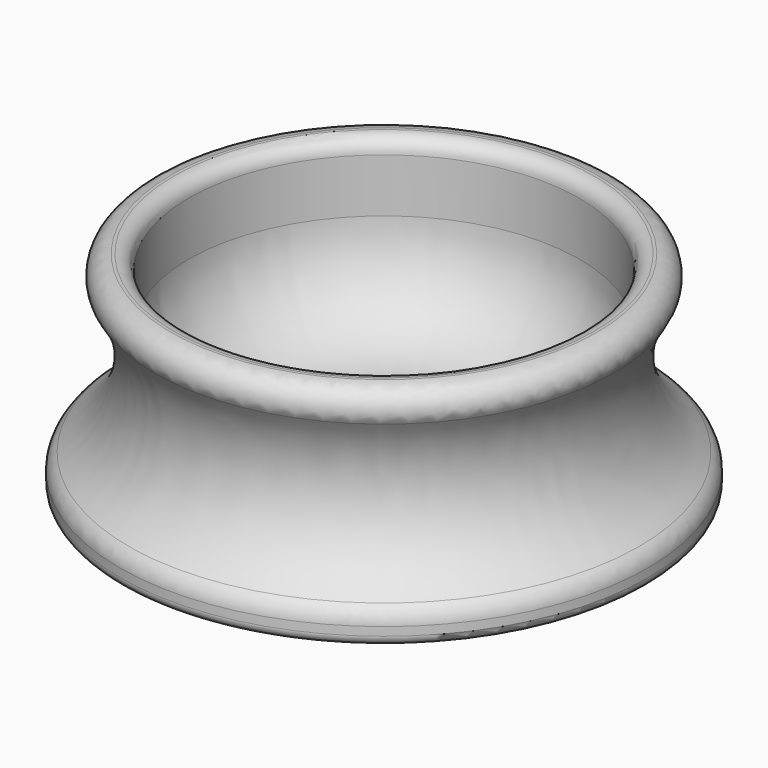
from build123d import *

# Parameters (mm, degrees)
F2_R     = 10
F3_R     = 2
F4_R     = 1.5
F5_W     = 10
F5_H     = 10
F6_DEPTH = 21.4010001
F7_R     = 1
F8_SIZE  = 1


with BuildPart() as f1:
    # F0 (on Front) → F1 (revolve)
    with BuildSketch(Plane.XZ):
        with BuildLine():
            ThreePointArc((-27, 18.4), (-21.5, 9.2), (-27, 0))
            Line((-27, 0), (-27, -3))
            Line((-27, -3), (0, -3))
            Line((0, -3), (0, 0))
            Line((0, 0), (0, 1.4))
            Line((0, 1.4), (-20, 1.4))
            Line((-20, 1.4), (-20, 18.4))
            Line((-20, 18.4), (-27, 18.4))
        make_face()
    revolve(axis=Axis((0, 0, 0.7), (0, 0, 1)))

    # F2
    f2_edges = [f1.edges().sort_by_distance(p)[0] for p in [
        (20, 0, 1.4),
    ]]
    fillet(f2_edges, radius=F2_R)

    # F3
    f3_edges = [f1.edges().sort_by_distance(p)[0] for p in [
        (27, 0, 18.4),
        (27, 0, 0),
    ]]
    fillet(f3_edges, radius=F3_R)

    # F4
    f4_edges = [f1.edges().sort_by_distance(p)[0] for p in [
        (20, 0, 18.4),
    ]]
    fillet(f4_edges, radius=F4_R)

    # F5 (on face) → F6 (cut, through all)
    with BuildSketch(Plane(origin=(0, 0, -3), x_dir=(1, 0, 0), z_dir=(0, 0, -1))):
        Rectangle(F5_W, F5_H)
    extrude(amount=-F6_DEPTH, mode=Mode.SUBTRACT)

    # F7
    f7_edges = [f1.edges().sort_by_distance(p)[0] for p in [
        (27, 0, -3),
    ]]
    fillet(f7_edges, radius=F7_R)

    # F8
    f8_edges = [f1.edges().sort_by_distance(p)[0] for p in [
        (5, 0, 1.4),
        (0, 5, 1.4),
        (-5, 0, 1.4),
        (0, -5, 1.4),
    ]]
    chamfer(f8_edges, length=F8_SIZE)


solid = f1.part
